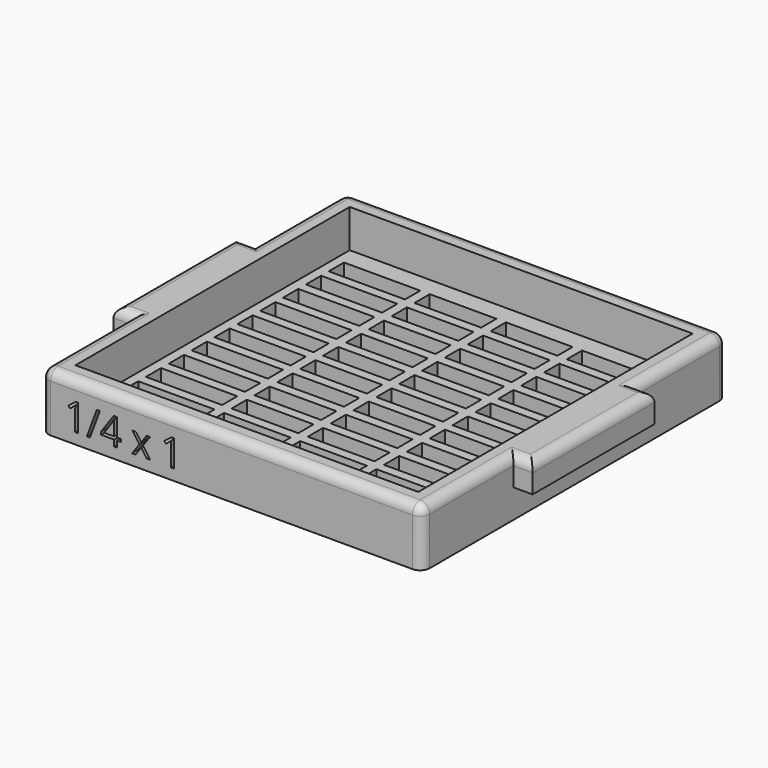
from build123d import *

# Parameters (mm, degrees)
F1_DEPTH     = 6.35
F0_W         = 6.35
F0_H         = 50.8
F2_DEPTH     = 19.05
F3_W         = 25.4
F3_H         = 6.35
F3_W_2       = 22.225
F4_DEPTH     = 25.4
F5_R         = 3.175
F6_W         = 6.35
F6_H         = 50.8
F7_DEPTH     = 9.525
F8_TEXT_SIZE = 12.4973367848
F9_DEPTH     = 3.175


# Not quite as in the source:
# - a feature names something its author has since deleted; it is built from what else it names
# - Text() gives the source's letters only with a copy of the font that has no kerning and outlines rounded to 1/6400 em; it was checked with that copy


with BuildPart() as f1:
    # F0 (on Top) → F1 (new body)
    with BuildSketch(Plane.XY):
        Polygon((-57.15, 25.1415750563), (-57.15, -25.6584249437), (-57.15, -57.4084249437), (57.15, -57.4084249437), (57.15, -25.6584249437), (57.15, 25.1415750563), (57.15, 56.8915750563), (-57.15, 56.8915750563), align=None)
    extrude(amount=F1_DEPTH)

    # F0 (on Top) → F2 (join)
    with BuildSketch(Plane.XY):
        Polygon((-63.5, -25.6584249437), (-63.5, -63.7584249437), (63.5, -63.7584249437), (63.5, -25.6584249437), (57.15, -25.6584249437), (57.15, -57.4084249437), (-57.15, -57.4084249437), (-57.15, -25.6584249437), align=None)
        with Locations((-66.675, -0.2584249437)):
            Rectangle(F0_W, F0_H)
        with Locations((-60.325, -0.2584249437)):
            Rectangle(F0_W, F0_H)
        with Locations((60.325, -0.2584249437)):
            Rectangle(F0_W, F0_H)
        with Locations((66.675, -0.2584249437)):
            Rectangle(F0_W, F0_H)
        Polygon((-63.5, 63.2415750563), (-63.5, 25.1415750563), (-57.15, 25.1415750563), (-57.15, 56.8915750563), (57.15, 56.8915750563), (57.15, 25.1415750563), (63.5, 25.1415750563), (63.5, 63.2415750563), align=None)
    extrude(amount=F2_DEPTH)

    # F3 (on face) → F4 (cut)
    with BuildSketch(Plane.XY.offset(6.35)):
        with Locations((-41.275, -47.8834249437)):
            Rectangle(F3_W, F3_H)
        with Locations((-41.275, -38.3584249437)):
            Rectangle(F3_W, F3_H)
        with Locations((-41.275, -28.8334249437)):
            Rectangle(F3_W, F3_H)
        with Locations((-41.275, -19.3084249437)):
            Rectangle(F3_W, F3_H)
        with Locations((-41.275, -9.7834249437)):
            Rectangle(F3_W, F3_H)
        with Locations((-41.275, -0.2584249437)):
            Rectangle(F3_W, F3_H)
        with Locations((-41.275, 9.2665750563)):
            Rectangle(F3_W, F3_H)
        with Locations((-41.275, 18.7915750563)):
            Rectangle(F3_W, F3_H)
        with Locations((-41.275, 28.3165750563)):
            Rectangle(F3_W, F3_H)
        with Locations((-41.275, 37.8415750563)):
            Rectangle(F3_W, F3_H)
        with Locations((-41.275, 47.3665750563)):
            Rectangle(F3_W, F3_H)
        with Locations((-14.2875, -47.8834249437)):
            Rectangle(F3_W_2, F3_H)
        with Locations((-14.2875, -38.3584249437)):
            Rectangle(F3_W_2, F3_H)
        with Locations((11.1125, -47.8834249437)):
            Rectangle(F3_W_2, F3_H)
        with Locations((11.1125, -38.3584249437)):
            Rectangle(F3_W_2, F3_H)
        with Locations((38.1, -47.8834249437)):
            Rectangle(F3_W, F3_H)
        with Locations((38.1, -38.3584249437)):
            Rectangle(F3_W, F3_H)
        with Locations((38.1, -28.8334249437)):
            Rectangle(F3_W, F3_H)
        with Locations((38.1, -19.3084249437)):
            Rectangle(F3_W, F3_H)
        with Locations((11.1125, -19.3084249437)):
            Rectangle(F3_W_2, F3_H)
        with Locations((11.1125, -28.8334249437)):
            Rectangle(F3_W_2, F3_H)
        with Locations((-14.2875, -28.8334249437)):
            Rectangle(F3_W_2, F3_H)
        with Locations((-14.2875, -19.3084249437)):
            Rectangle(F3_W_2, F3_H)
        with Locations((38.1, -9.7834249437)):
            Rectangle(F3_W, F3_H)
        with Locations((38.1, -0.2584249437)):
            Rectangle(F3_W, F3_H)
        with Locations((38.1, 9.2665750563)):
            Rectangle(F3_W, F3_H)
        with Locations((11.1125, -9.7834249437)):
            Rectangle(F3_W_2, F3_H)
        with Locations((11.1125, -0.2584249437)):
            Rectangle(F3_W_2, F3_H)
        with Locations((11.1125, 9.2665750563)):
            Rectangle(F3_W_2, F3_H)
        with Locations((-14.2875, -9.7834249437)):
            Rectangle(F3_W_2, F3_H)
        with Locations((-14.2875, -0.2584249437)):
            Rectangle(F3_W_2, F3_H)
        with Locations((-14.2875, 9.2665750563)):
            Rectangle(F3_W_2, F3_H)
        with Locations((-14.2875, 18.7915750563)):
            Rectangle(F3_W_2, F3_H)
        with Locations((-14.2875, 28.3165750563)):
            Rectangle(F3_W_2, F3_H)
        with Locations((-14.2875, 37.8415750563)):
            Rectangle(F3_W_2, F3_H)
        with Locations((-14.2875, 47.3665750563)):
            Rectangle(F3_W_2, F3_H)
        with Locations((11.1125, 18.7915750563)):
            Rectangle(F3_W_2, F3_H)
        with Locations((11.1125, 28.3165750563)):
            Rectangle(F3_W_2, F3_H)
        with Locations((11.1125, 37.8415750563)):
            Rectangle(F3_W_2, F3_H)
        with Locations((11.1125, 47.3665750563)):
            Rectangle(F3_W_2, F3_H)
        with Locations((38.1, 47.3665750563)):
            Rectangle(F3_W, F3_H)
        with Locations((38.1, 37.8415750563)):
            Rectangle(F3_W, F3_H)
        with Locations((38.1, 28.3165750563)):
            Rectangle(F3_W, F3_H)
        with Locations((38.1, 18.7915750563)):
            Rectangle(F3_W, F3_H)
    extrude(amount=-F4_DEPTH, mode=Mode.SUBTRACT)

    # F5
    f5_edges = [f1.edges().sort_by_distance(p)[0] for p in [
        (-63.5, -44.708425, 19.05),
        (0, -63.758425, 19.05),
        (63.5, -44.708425, 19.05),
        (66.675, -25.658425, 19.05),
        (69.85, -0.258425, 19.05),
        (-66.675, -25.658425, 19.05),
        (-69.85, -0.258425, 19.05),
        (-66.675, 25.141575, 19.05),
        (-63.5, 44.191575, 19.05),
        (0, 63.241575, 19.05),
        (63.5, 44.191575, 19.05),
        (66.675, 25.141575, 19.05),
        (63.5, -63.758425, 9.525),
        (-63.5, -63.758425, 9.525),
        (-63.5, 63.241575, 9.525),
        (63.5, 63.241575, 9.525),
    ]]
    fillet(f5_edges, radius=F5_R)

    # F6 (on face) → F7 (cut)
    with BuildSketch(Plane(origin=(0, 0, 0), x_dir=(1, 0, 0), z_dir=(0, 0, -1))):
        with Locations((-66.675, 0.2584249437)):
            Rectangle(F6_W, F6_H)
        with Locations((66.675, 0.2584249437)):
            Rectangle(F6_W, F6_H)
    extrude(amount=-F7_DEPTH, mode=Mode.SUBTRACT)

    # F8 (on face) → F9 (cut)
    with BuildSketch(Plane.XZ.offset(63.7584249437)):
        with Locations((-55.5181726813, 3.6184177734)):
            Text('1/4 x 1', F8_TEXT_SIZE, font='Open Sans', text_align=(TextAlign.LEFT, TextAlign.BOTTOM))
    extrude(amount=-F9_DEPTH, mode=Mode.SUBTRACT)


solid = f1.part
